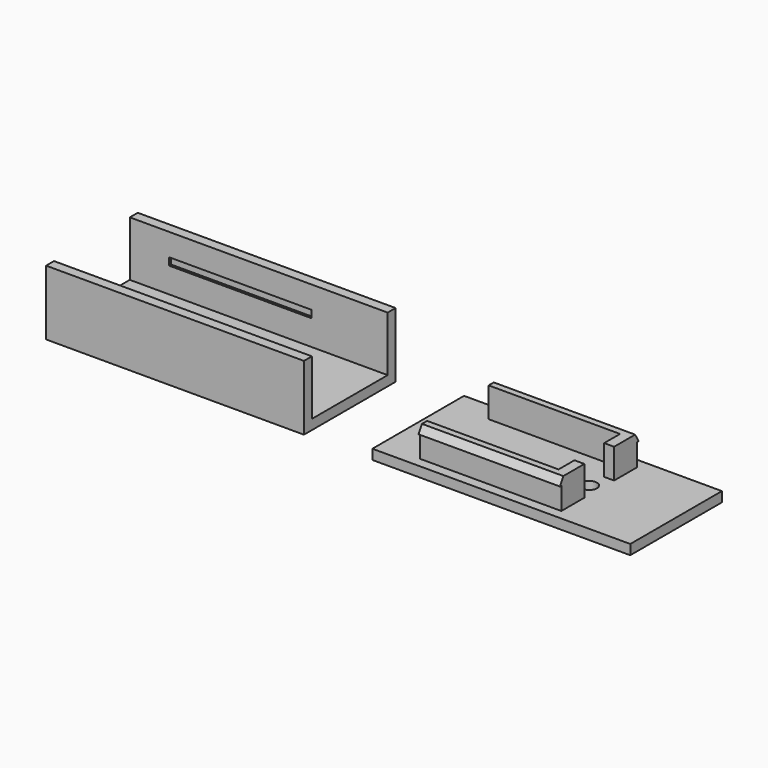
from build123d import *

# Parameters (mm, degrees)
F0_W         = 52
F0_H         = 23.1
F1_DEPTH     = 2
F3_W         = 52
F3_H         = 2
F4_DEPTH     = 11.1
F5_W         = 28.5
F5_H         = 1.8
F6_DEPTH     = 6
F7_W         = 28.5
F7_H         = 1.5
F8_DEPTH     = 0.5
F9_T1_DEPTH  = 37.4619279412
F10_W        = 28.5
F10_H        = 1.5
F11_DEPTH    = 0.5
F12_T1_DEPTH = 37.4619279412
F13_W        = 28.7
F13_H        = 1.5
F14_DEPTH    = 0.5
F15_W        = 28.7
F15_H        = 1.5
F16_DEPTH    = 0.5
F17_R        = 1.55
F18_DEPTH    = 2.001
F19_W        = 2
F19_H        = 4
F20_DEPTH    = 6


# Not quite as in the source:
# - a fillet or chamfer that OpenCascade refuses, or shapes differently, is made with other operations: its cross-section is extruded or revolved along the edge and cut away or added


with BuildPart() as f1:
    # F0 (on Top) → F1 (new body)
    with BuildSketch(Plane.XY):
        Rectangle(F0_W, F0_H)
    extrude(amount=F1_DEPTH)


with BuildPart() as f2_1:
    # F2: copy of F1
    add(f1.part.moved(Location((65.8, 0, 0))))

    # F5 (on face) → F6 (join)
    with BuildSketch(Plane.XY.offset(2)):
        with Locations((62.05, -8.65)):
            Rectangle(F5_W, F5_H)
        with Locations((62.05, 8.65)):
            Rectangle(F5_W, F5_H)
    extrude(amount=F6_DEPTH)

    # F7 (on face) → F8 (join)
    with BuildSketch(Plane.XZ.offset(9.55)):
        with Locations((62.05, 7.25)):
            Rectangle(F7_W, F7_H)
    extrude(amount=F8_DEPTH)

    # F9: chamfer of 1 x 1.7320508076 on 1 edges, made by hand

    # F9_s2 → F9_t1 (cut)
    with BuildSketch(Plane.YZ.offset(43.3190360294)):
        Polygon((-9.05, 8), (-10.05, 6.2679491924), (-10.05, 8), align=None)
    extrude(amount=F9_T1_DEPTH, mode=Mode.SUBTRACT)

    # F10 (on face) → F11 (join)
    with BuildSketch(Plane(origin=(0, 9.55, 0), x_dir=(-1, 0, 0), z_dir=(0, 1, 0))):
        with Locations((-62.05, 7.25)):
            Rectangle(F10_W, F10_H)
    extrude(amount=F11_DEPTH)

    # F12: chamfer of 1 x 1.7320508076 on 1 edges, made by hand

    # F12_s2 → F12_t1 (cut)
    with BuildSketch(Plane.YZ.offset(43.3190360294)):
        Polygon((10.05, 6.2679491924), (9.05, 8), (10.05, 8), align=None)
    extrude(amount=F12_T1_DEPTH, mode=Mode.SUBTRACT)

    # F17 (on face) → F18 (cut, through all)
    with BuildSketch(Plane.XY.offset(2)):
        with Locations((74.3, 0)):
            Circle(F17_R)
    extrude(amount=-F18_DEPTH, mode=Mode.SUBTRACT)

    # F19 (on face) → F20 (join)
    with BuildSketch(Plane.XY.offset(2)):
        with Locations((75.3, -5.75)):
            Rectangle(F19_W, F19_H)
        with Locations((75.3, 5.75)):
            Rectangle(F19_W, F19_H)
    extrude(amount=F20_DEPTH)


with BuildPart() as f1_1:
    add(f1.part)

    # F3 (on face) → F4 (join)
    with BuildSketch(Plane.XY.offset(2)):
        with Locations((0, -10.55)):
            Rectangle(F3_W, F3_H)
        with Locations((0, 10.55)):
            Rectangle(F3_W, F3_H)
    extrude(amount=F4_DEPTH)

    # F13 (on face) → F14 (cut)
    with BuildSketch(Plane(origin=(0, -9.55, 0), x_dir=(-1, 0, 0), z_dir=(0, 1, 0))):
        with Locations((3.75, 7.85)):
            Rectangle(F13_W, F13_H)
    extrude(amount=-F14_DEPTH, mode=Mode.SUBTRACT)

    # F15 (on face) → F16 (cut)
    with BuildSketch(Plane.XZ.offset(-9.55)):
        with Locations((-3.75, 7.85)):
            Rectangle(F15_W, F15_H)
    extrude(amount=-F16_DEPTH, mode=Mode.SUBTRACT)


solid = Compound([f2_1.part, f1_1.part])
